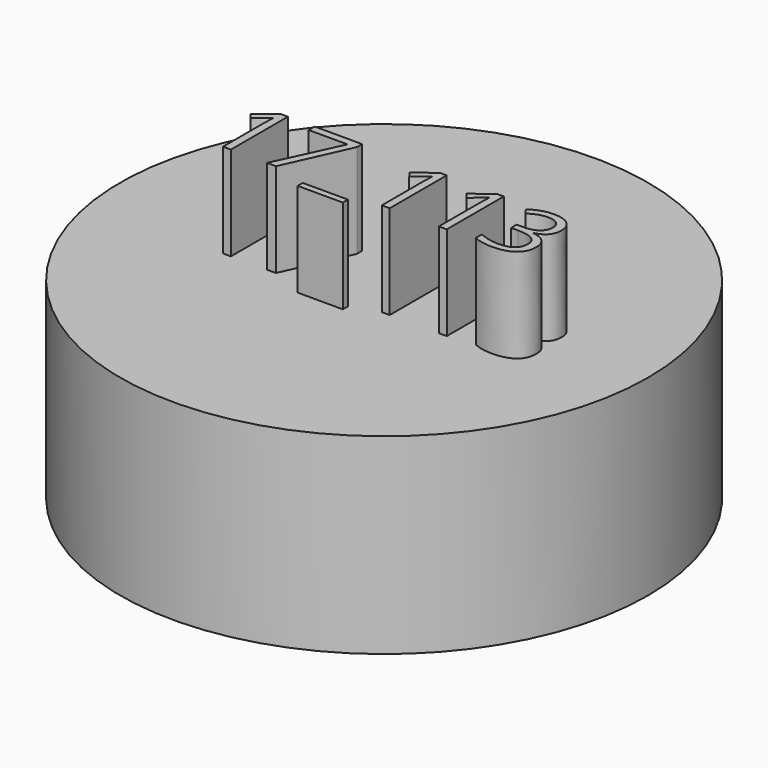
from build123d import *

# Parameters (mm, degrees)
F0_R         = 71.3205808401
F1_DEPTH     = 51.816
F2_TEXT_SIZE = 26.9610861627
F3_DEPTH     = 25.4


# Not quite as in the source:
# - Text() gives the source's letters only with a copy of the font that has no kerning and outlines rounded to 1/6400 em; it was checked with that copy


with BuildPart() as f1:
    # F0 (on Top) → F1 (new body)
    with BuildSketch(Plane.XY):
        Circle(F0_R)
    extrude(amount=F1_DEPTH)

    # F2 (on face) → F3 (join)
    with BuildSketch(Plane.XY.offset(51.816)):
        with Locations((-41.4430387318, -11.7088063271)):
            Text('17_113', F2_TEXT_SIZE, font='Open Sans', text_align=(TextAlign.LEFT, TextAlign.BOTTOM))
    extrude(amount=F3_DEPTH)


solid = f1.part
